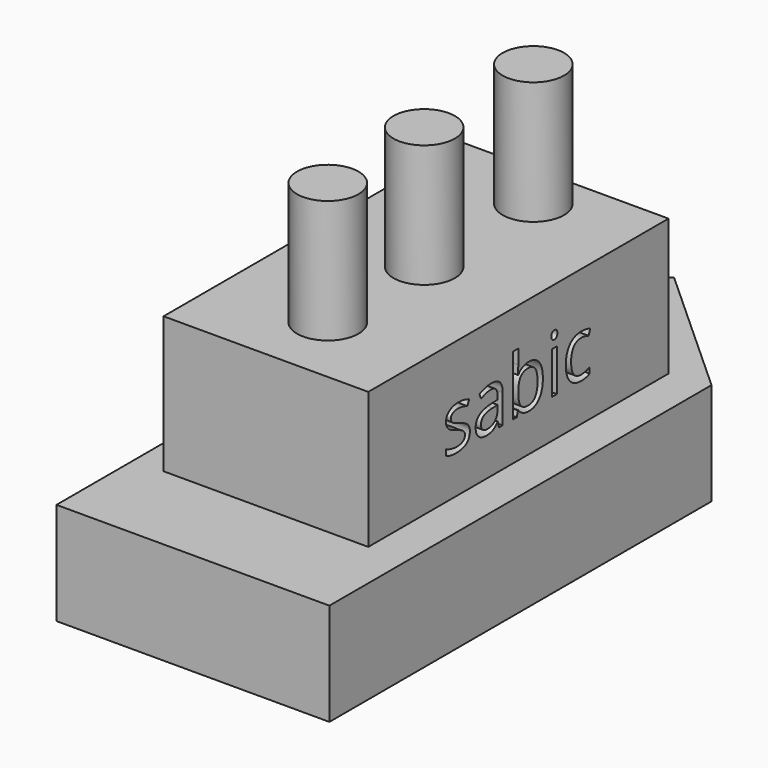
from build123d import *

# Parameters (mm, degrees)
F1_DEPTH     = 15
F2_W         = 30
F2_H         = 55
F3_DEPTH     = 20
F4_R         = 4.5
F5_DEPTH     = 18
F6_TEXT_SIZE = 11.5343317803
F7_DEPTH     = 34.3774822226


# Not quite as in the source:
# - Text() gives the source's letters only with a copy of the font that has no kerning and outlines rounded to 1/6400 em; it was checked with that copy


with BuildPart() as f1:
    # F0 (on Top) → F1 (new body)
    with BuildSketch(Plane.XY):
        Polygon((20, 20), (0, 38.1383571472), (-20, 20), (-20, -50), (20, -50), align=None)
    extrude(amount=F1_DEPTH)

    # F2 (on face) → F3 (join)
    with BuildSketch(Plane.XY.offset(15)):
        with Locations((-0.6235177774, -8.3508552313)):
            Rectangle(F2_W, F2_H)
    extrude(amount=F3_DEPTH)

    # F4 (on face) → F5 (join)
    with BuildSketch(Plane.XY.offset(35)):
        with Locations((0, 12.3599059247)):
            Circle(F4_R)
        with Locations((0, -7.6400940753)):
            Circle(F4_R)
        with Locations((0, -25.2996686119)):
            Circle(F4_R)
    extrude(amount=F5_DEPTH)

    # F6 (on face) → F7 (cut, through all)
    with BuildSketch(Plane.YZ.offset(14.3764822226)):
        with Locations((-22.2113449126, 20.6658653915)):
            Text('sabic', F6_TEXT_SIZE, font='Open Sans', text_align=(TextAlign.LEFT, TextAlign.BOTTOM))
    extrude(amount=-F7_DEPTH, mode=Mode.SUBTRACT)


solid = f1.part
